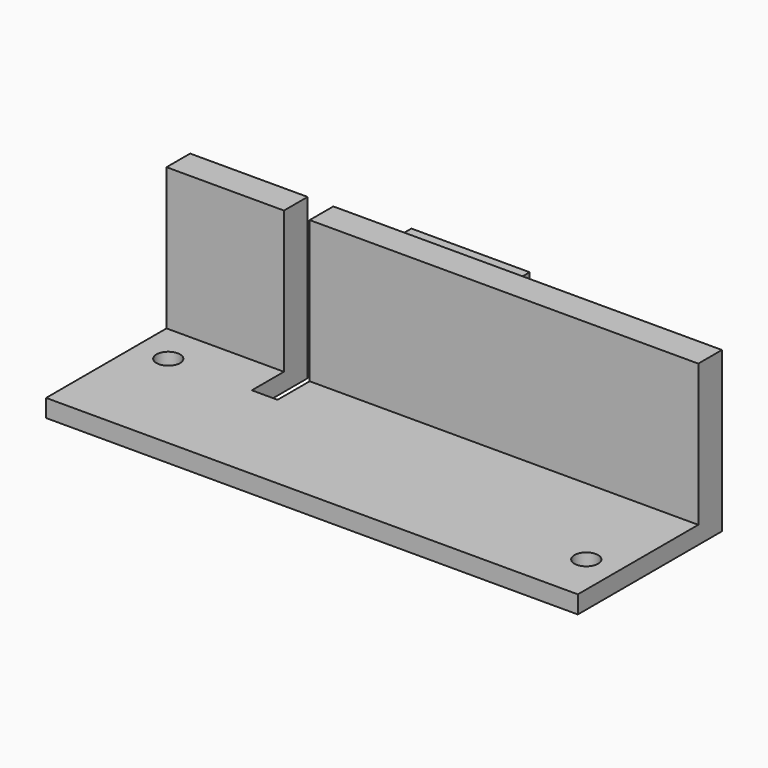
from build123d import *

# Parameters (mm, degrees)
F0_R     = 2
F1_DEPTH = 3
F2_W     = 19.86
F2_H     = 24
F2_H_2   = 3
F3_DEPTH = 3
F4_W     = 20
F4_H     = 2.75
F5_DEPTH = 2.75
F6_W     = 20
F6_H     = 1.9
F7_DEPTH = 1.9
F8_DEPTH = 2


with BuildPart() as f1:
    # F0 (on Top) → F1 (new body)
    with BuildSketch(Plane.XY):
        Polygon((-44.965, -13.73), (44.965, -13.73), (44.965, 13.73), (-20.755, 13.73), (-20.755, 4.94), (-25.105, 4.94), (-25.105, 13.73), (-44.965, 13.73), align=None)
        with Locations((39.595, -5.23)):
            Circle(F0_R, mode=Mode.SUBTRACT)
        with Locations((-39.365, 5.1)):
            Circle(F0_R, mode=Mode.SUBTRACT)
    extrude(amount=F1_DEPTH)

    # F2 (on face) → F3 (join)
    with BuildSketch(Plane(origin=(0, 13.73, 0), x_dir=(-1, 0, 0), z_dir=(0, 1, 0))):
        Polygon((11.269, 0), (20.755, 0), (20.755, 3), (20.755, 27), (-44.965, 27), (-44.965, 3), (-44.965, 0), (-8.731, 0), align=None)
        with Locations((35.035, 15)):
            Rectangle(F2_W, F2_H)
        with Locations((35.035, 1.5)):
            Rectangle(F2_W, F2_H_2)
    extrude(amount=F3_DEPTH)

    # F4 (on face) → F5 (join)
    with BuildSketch(Plane(origin=(0, 16.73, 0), x_dir=(-1, 0, 0), z_dir=(0, 1, 0))):
        with Locations((1.269, 21.625)):
            Rectangle(F4_W, F4_H)
    extrude(amount=F5_DEPTH)

    # F6 (on face) → F7 (join)
    with BuildSketch(Plane(origin=(0, 19.48, 0), x_dir=(-1, 0, 0), z_dir=(0, 1, 0))):
        Polygon((11.269, 20.25), (-8.731, 20.25), (-8.731, 18.5663476586), (-4.159652628, 18.27), (0.319, 18.27), (0.519, 19.52), (4.269, 19.52), (4.269, 18.27), (11.269, 18.27), align=None)
        Polygon((-8.731, 23), (-8.731, 20.25), (11.269, 20.25), (11.269, 21.625), (11.269, 23), align=None)
        with Locations((1.269, 23.95)):
            Rectangle(F6_W, F6_H)
    extrude(amount=F7_DEPTH)

    # F2 (on face) → F8 (join)
    with BuildSketch(Plane(origin=(0, 13.73, 0), x_dir=(-1, 0, 0), z_dir=(0, 1, 0))):
        with Locations((35.035, 15)):
            Rectangle(F2_W, F2_H)
        Polygon((11.269, 0), (20.755, 0), (20.755, 3), (20.755, 27), (-44.965, 27), (-44.965, 3), (-44.965, 0), (-8.731, 0), align=None)
    extrude(amount=-F8_DEPTH)


solid = f1.part
